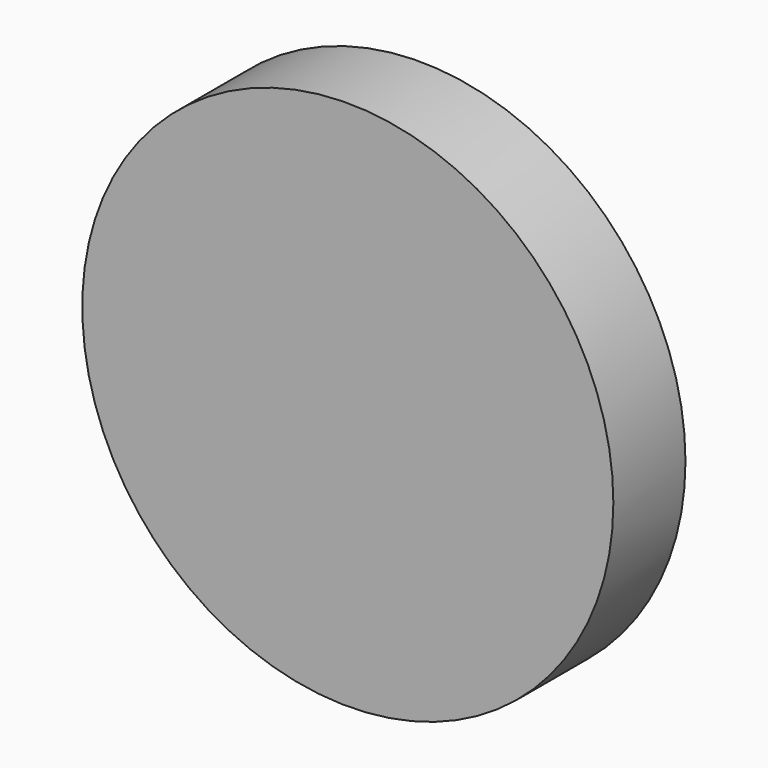
from build123d import *

# Parameters (mm, degrees)
F0_R     = 88.3698573987
F1_DEPTH = 30


# Not quite as in the source:
# - the program builds the solid bodies; features that only make, move or delete a surface that nothing else refers to are left out


with BuildPart() as f1:
    # F0 (on Front) → F1 (new body)
    with BuildSketch(Plane.XZ):
        Circle(F0_R)
    extrude(amount=F1_DEPTH)


solid = f1.part
